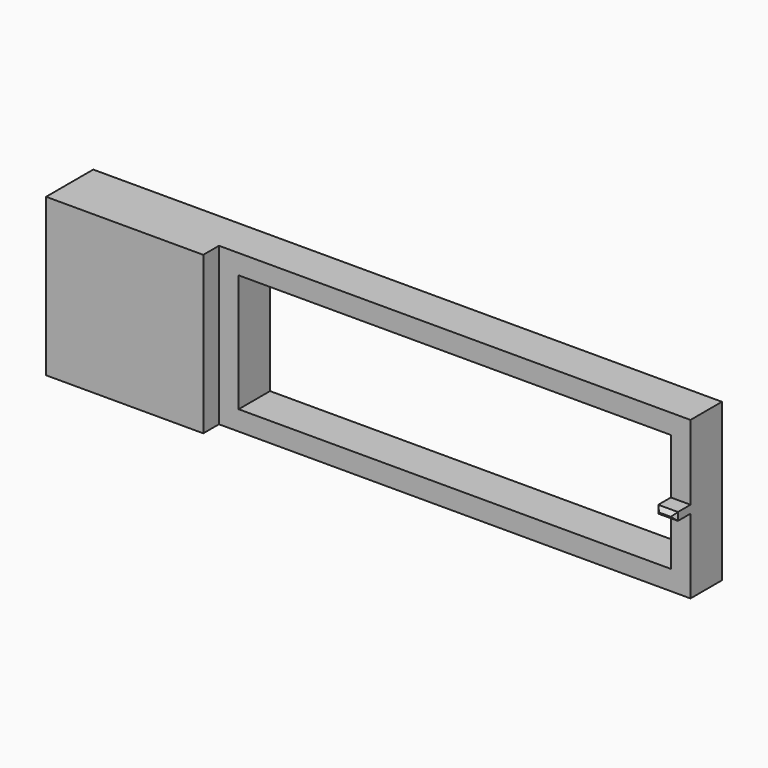
from build123d import *

# Parameters (mm, degrees)
F0_W     = 12.7
F0_H     = 12.7
F1_DEPTH = 4.7625
F2_W     = 38.1
F2_H     = 12.7
F2_W_2   = 34.925
F2_H_2   = 9.525
F3_DEPTH = 3.175
F4_W     = 1.5875
F4_H     = 0.635
F5_DEPTH = 1.5875
F6_SIZE  = 0.31749


# Not quite as in the source:
# - a fillet or chamfer is up to 0.001 mm smaller than in the source, because OpenCascade refuses the exact size


with BuildPart() as f1:
    # F0 (on Front) → F1 (new body)
    with BuildSketch(Plane.XZ):
        Rectangle(F0_W, F0_H)
    extrude(amount=F1_DEPTH)

    # F2 (on Front) → F3 (join)
    with BuildSketch(Plane.XZ):
        with Locations((25.4, 0)):
            Rectangle(F2_W, F2_H)
        with Locations((25.4, 0)):
            Rectangle(F2_W_2, F2_H_2, mode=Mode.SUBTRACT)
    extrude(amount=F3_DEPTH)

    # F4 (on face) → F5 (join)
    with BuildSketch(Plane.XZ.offset(3.175)):
        with Locations((43.65625, 0)):
            Rectangle(F4_W, F4_H)
    extrude(amount=F5_DEPTH)

    # F6 (size 0.3175 in the source; OpenCascade refuses exactly that, so slightly less here)
    f6_edges = [f1.edges().sort_by_distance(p)[0] for p in [
        (43.65625, -4.7625, 0.3175),
        (42.8625, -4.7625, 0),
        (43.65625, -4.7625, -0.3175),
        (44.45, -4.7625, 0),
    ]]
    chamfer(f6_edges, length=F6_SIZE)


solid = f1.part
